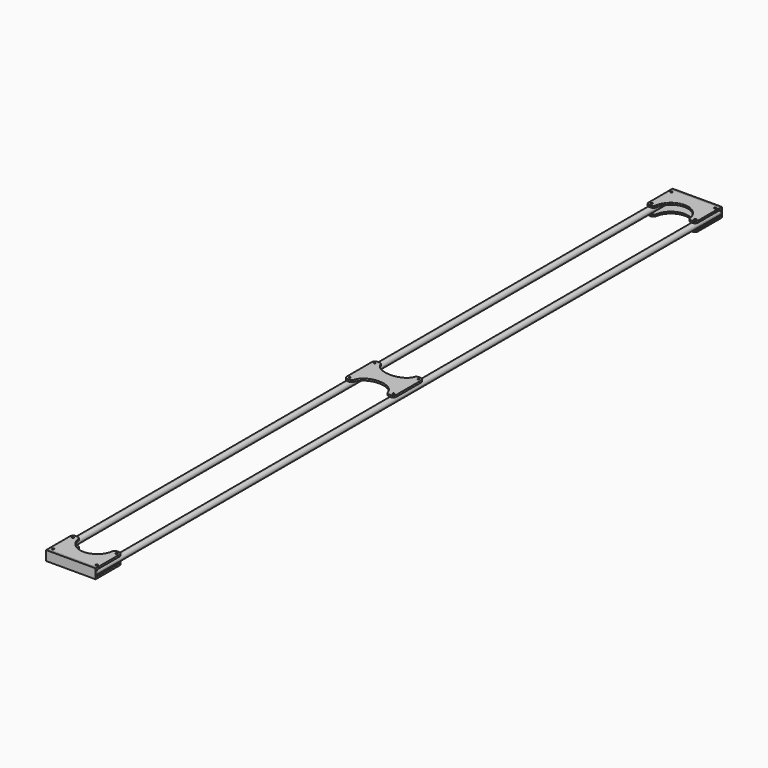
from build123d import *

# Parameters (mm, degrees)
F0_R          = 9.5
F0_R_2        = 9
F1_DEPTH      = 1250
F5_DEPTH      = 6
F6_R          = 10
F7_R          = 2.5
F8_DEPTH      = 6.0010001
F8_DEPTH_BACK = 5
F10_DEPTH     = 6
F11_R         = 10
F13_R         = 3.175
F14_DEPTH     = 31.001
F16_W         = 159
F16_H         = 31
F17_DEPTH     = 6
F19_R         = 4.5
F20_DEPTH     = 15.501
F21_R         = 1
F21_2_R       = 1
F21_3_R       = 1


with BuildPart() as f1:
    # F0 (on Front) → F1 (new body, symmetric)
    with BuildSketch(Plane.XZ):
        with Locations((-70, 0)):
            Circle(F0_R)
        with Locations((-70, 0)):
            Circle(F0_R_2, mode=Mode.SUBTRACT)
    extrude(amount=F1_DEPTH, both=True)


with BuildPart() as f2_1:
    # F2: instance of F1
    add(f1.part.mirror(Plane.YZ))


with BuildPart() as f5:
    # F4 (on offset) → F5 (new body)
    with BuildSketch(Plane.XY.offset(9.5)):
        with BuildLine():
            Line((-55, 60), (-79.5, 60))
            Line((-79.5, 60), (-79.5, -60))
            Line((-79.5, -60), (-55, -60))
            add(Edge.make_bspline(
                [(55, -60), (55, -20), (0, -20), (-55, -20), (-55, -60)],
                knots=[3.1415926536, 3.1415926536, 3.1415926536, 4.7123889804, 4.7123889804, 6.2831853072, 6.2831853072, 6.2831853072], degree=2, weights=[1, 0.7071067812, 1, 0.7071067812, 1]))
            Line((55, -60), (79.5, -60))
            Line((79.5, -60), (79.5, 60))
            Line((79.5, 60), (55, 60))
            add(Edge.make_bspline(
                [(-55, 60), (-55, 25), (0, 25), (55, 25), (55, 60)],
                knots=[0, 0, 0, 1.5707963268, 1.5707963268, 3.1415926536, 3.1415926536, 3.1415926536], degree=2, weights=[1, 0.7071067812, 1, 0.7071067812, 1]))
        make_face()
    extrude(amount=F5_DEPTH)

    # F6
    f6_edges = [f5.edges().sort_by_distance(p)[0] for p in [
        (-79.5, 60, 12.5),
        (-79.5, -60, 12.5),
        (-55, -60, 12.5),
        (55, -60, 12.5),
        (79.5, -60, 12.5),
        (55, 60, 12.5),
        (79.5, 60, 12.5),
        (-55, 60, 12.5),
    ]]
    fillet(f6_edges, radius=F6_R)


with BuildPart() as f8_tool:
    # F7 (on offset) → F8 (new body, two sides)
    with BuildSketch(Plane.XY.offset(9.5)) as f8_sk:
        with Locations((-70, 50)):
            Circle(F7_R)
        with Locations((70, 50)):
            Circle(F7_R)
        with Locations((70, -50)):
            Circle(F7_R)
        with Locations((-70, -50)):
            Circle(F7_R)
    extrude(amount=F8_DEPTH)
    extrude(f8_sk.sketch, amount=-F8_DEPTH_BACK)


with BuildPart() as f1_1:
    add(f1.part)

    # F8: cut by f8_tool
    add(f8_tool.part, mode=Mode.SUBTRACT)


with BuildPart() as f5_1:
    add(f5.part)

    # F8: cut by f8_tool
    add(f8_tool.part, mode=Mode.SUBTRACT)


with BuildPart() as f10:
    # F9 (on offset) → F10 (new body)
    with BuildSketch(Plane.XY.offset(9.5)):
        with BuildLine():
            Line((-79.5, -1150), (-79.5, -1250))
            Line((-79.5, -1250), (79.5, -1250))
            Line((79.5, -1250), (79.5, -1150))
            Line((79.5, -1150), (55, -1150))
            ThreePointArc((55, -1150), (0, -1205), (-55, -1150))
            Line((-55, -1150), (-79.5, -1150))
        make_face()
    extrude(amount=F10_DEPTH)

    # F11
    f11_edges = [f10.edges().sort_by_distance(p)[0] for p in [
        (-79.5, -1150, 12.5),
        (-55, -1150, 12.5),
        (55, -1150, 12.5),
        (79.5, -1150, 12.5),
    ]]
    fillet(f11_edges, radius=F11_R)


with BuildPart() as f12_1:
    # F12: instance of F10
    add(f10.part.mirror(Plane.XY))


with BuildPart() as f14_tool:
    # F13 (on face) → F14 (new body, through all)
    with BuildSketch(Plane.XY.offset(15.5)):
        with Locations((-70, -1160)):
            Circle(F13_R)
        with Locations((70, -1160)):
            Circle(F13_R)
        with Locations((70, -1240)):
            Circle(F13_R)
        with Locations((-70, -1240)):
            Circle(F13_R)
    extrude(amount=-F14_DEPTH)


with BuildPart() as f1_2:
    add(f1_1.part)

    # F14: cut by f14_tool
    add(f14_tool.part, mode=Mode.SUBTRACT)


with BuildPart() as f10_1:
    add(f10.part)

    # F14: cut by f14_tool
    add(f14_tool.part, mode=Mode.SUBTRACT)


with BuildPart() as f12_1_1:
    add(f12_1.part)

    # F14: cut by f14_tool
    add(f14_tool.part, mode=Mode.SUBTRACT)


with BuildPart() as f15_1:
    # F15: instance of F10
    add(f10_1.part.mirror(Plane.XZ))

    # F21
    f21_edges = [f15_1.edges().sort_by_distance(p)[0] for p in [
        (-79.5, 1205, 15.5),
        (-66.863081, 1150, 15.5),
        (-57.721727, 1152.404455, 15.5),
        (-76.571068, 1152.928932, 15.5),
        (0, 1205, 15.5),
        (57.721727, 1152.404455, 15.5),
        (66.863081, 1150, 15.5),
        (79.5, 1205, 15.5),
        (76.571068, 1152.928932, 15.5),
    ]]
    fillet(f21_edges, radius=F21_R)


with BuildPart() as f15_2:
    # F15: instance of F12_1
    add(f12_1_1.part.mirror(Plane.XZ))

    # F21#2
    f21_2_edges = [f15_2.edges().sort_by_distance(p)[0] for p in [
        (-79.5, 1205, -15.5),
        (-66.863081, 1150, -15.5),
        (-57.721727, 1152.404455, -15.5),
        (-76.571068, 1152.928932, -15.5),
        (0, 1205, -15.5),
        (57.721727, 1152.404455, -15.5),
        (66.863081, 1150, -15.5),
        (79.5, 1205, -15.5),
        (76.571068, 1152.928932, -15.5),
    ]]
    fillet(f21_2_edges, radius=F21_2_R)


with BuildPart() as f17:
    # F16 (on face) → F17 (new body)
    with BuildSketch(Plane.XZ.offset(1250)):
        Rectangle(F16_W, F16_H)
    extrude(amount=F17_DEPTH)


with BuildPart() as f18_1:
    # F18: instance of F17
    add(f17.part.mirror(Plane.XZ))

    # F21#3
    f21_3_edges = [f18_1.edges().sort_by_distance(p)[0] for p in [
        (-79.5, 1253, -15.5),
        (0, 1256, -15.5),
        (79.5, 1253, -15.5),
        (-79.5, 1256, 0),
        (-79.5, 1253, 15.5),
        (0, 1256, 15.5),
        (79.5, 1256, 0),
        (79.5, 1253, 15.5),
    ]]
    fillet(f21_3_edges, radius=F21_3_R)


with BuildPart() as f20_tool:
    # F19 (on Top) → F20 (new body, through all)
    with BuildSketch(Plane.XY):
        with Locations((70, 50)):
            Circle(F19_R)
        with Locations((70, -50)):
            Circle(F19_R)
        with Locations((-70, -50)):
            Circle(F19_R)
        with Locations((-70, 50)):
            Circle(F19_R)
    extrude(amount=-F20_DEPTH)


with BuildPart() as f1_3:
    add(f1_2.part)

    # F20: cut by f20_tool
    add(f20_tool.part, mode=Mode.SUBTRACT)


with BuildPart() as f2_1_1:
    add(f2_1.part)

    # F20: cut by f20_tool
    add(f20_tool.part, mode=Mode.SUBTRACT)


solid = Compound([f5_1.part, f10_1.part, f12_1_1.part, f15_1.part, f15_2.part, f17.part, f18_1.part, f1_3.part, f2_1_1.part])
